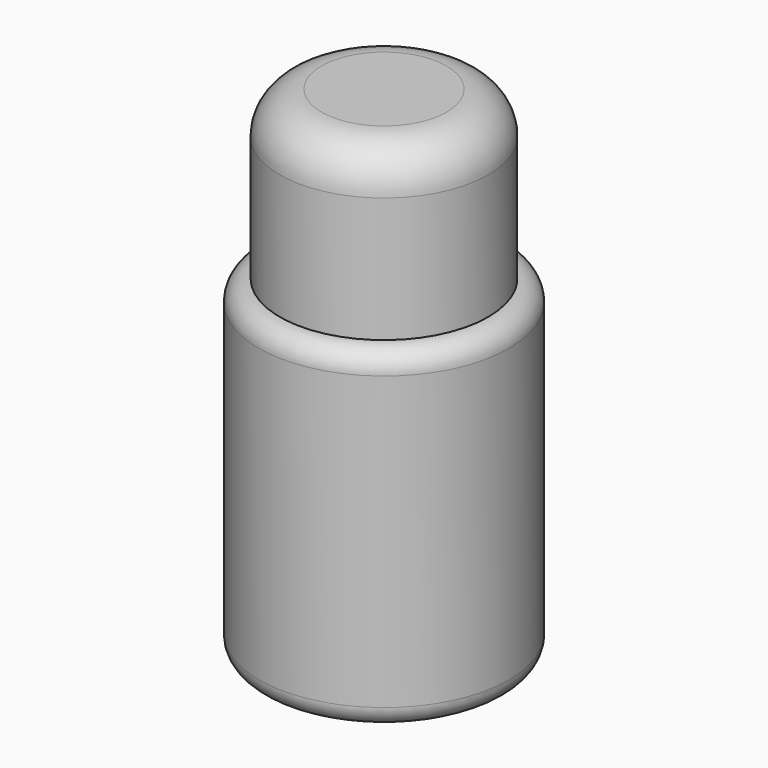
from build123d import *

# Parameters (mm, degrees)
F0_R     = 30
F1_DEPTH = 80
F2_R     = 25
F3_DEPTH = 40
F4_R     = 4.99999
F5_R     = 5
F6_R     = 10


# Not quite as in the source:
# - a fillet or chamfer is up to 0.001 mm smaller than in the source, because OpenCascade refuses the exact size


with BuildPart() as f1:
    # F0 (on Top) → F1 (new body)
    with BuildSketch(Plane.XY):
        Circle(F0_R)
    extrude(amount=F1_DEPTH)

    # F2 (on face) → F3 (join)
    with BuildSketch(Plane.XY.offset(80)):
        Circle(F2_R)
    extrude(amount=F3_DEPTH)

    # F4 (radius 5 in the source; OpenCascade refuses exactly that, so slightly less here)
    f4_edges = [f1.edges().sort_by_distance(p)[0] for p in [
        (-30, 0, 80),
    ]]
    fillet(f4_edges, radius=F4_R)

    # F5
    f5_edges = [f1.edges().sort_by_distance(p)[0] for p in [
        (-30, 0, 0),
    ]]
    fillet(f5_edges, radius=F5_R)

    # F6
    f6_edges = [f1.edges().sort_by_distance(p)[0] for p in [
        (-25, 0, 120),
    ]]
    fillet(f6_edges, radius=F6_R)


solid = f1.part
